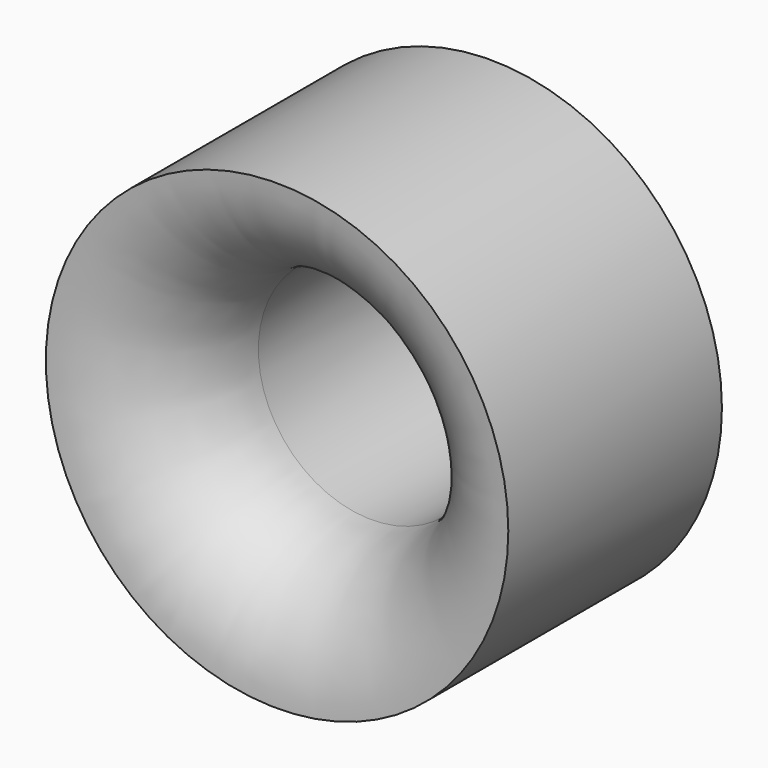
from build123d import *

# Parameters (mm, degrees)
F2_T = -5


# Not quite as in the source:
# - a fillet or chamfer that OpenCascade refuses, or shapes differently, is made with other operations: its cross-section is extruded or revolved along the edge and cut away or added


with BuildPart() as f1:
    # F0 (on Top) → F1 (revolve)
    with BuildSketch(Plane.XY):
        Polygon((0, 11.3076803427), (0, -11.3076803427), (9.7927384347, -5.6538401714), (9.7927384347, 5.6538401714), align=None)
    revolve(axis=Axis((0, 0, 0), (0, -1, 0)))

    # F2
    f2_openings = [f1.faces().sort_by_distance(p)[0] for p in [
        (-4.896369, -8.48076, 0),
        (-4.896369, 8.48076, 0),
    ]]
    offset(amount=F2_T, openings=f2_openings)

    # F3: fillet of radius 5 on 1 edges, made by hand

    # F3_s1 → F3_t2 (revolve, cut)
    with BuildSketch(Plane.XY):
        with BuildLine():
            ThreePointArc((9.7927384347, -5.6538401714), (6.2572045287, -4.1893740773), (4.7927384347, -0.6538401714))
            Line((4.7927384347, -0.6538401714), (4.6927384347, -0.6538401714))
            Line((4.6927384347, -0.6538401714), (4.6927384347, -8.5405915173))
            Line((4.6927384347, -8.5405915173), (4.8427384347, -8.6271940577))
            ThreePointArc((4.8427384347, -8.6271940577), (7.3427384347, -7.1838183847), (9.7927384347, -5.7538401714))
            Line((9.7927384347, -5.7538401714), (9.7927384347, -5.6538401714))
        make_face()
    revolve(axis=Axis((0, -8.5405915173, 0), (0, 1, 0)), mode=Mode.SUBTRACT)


solid = f1.part
